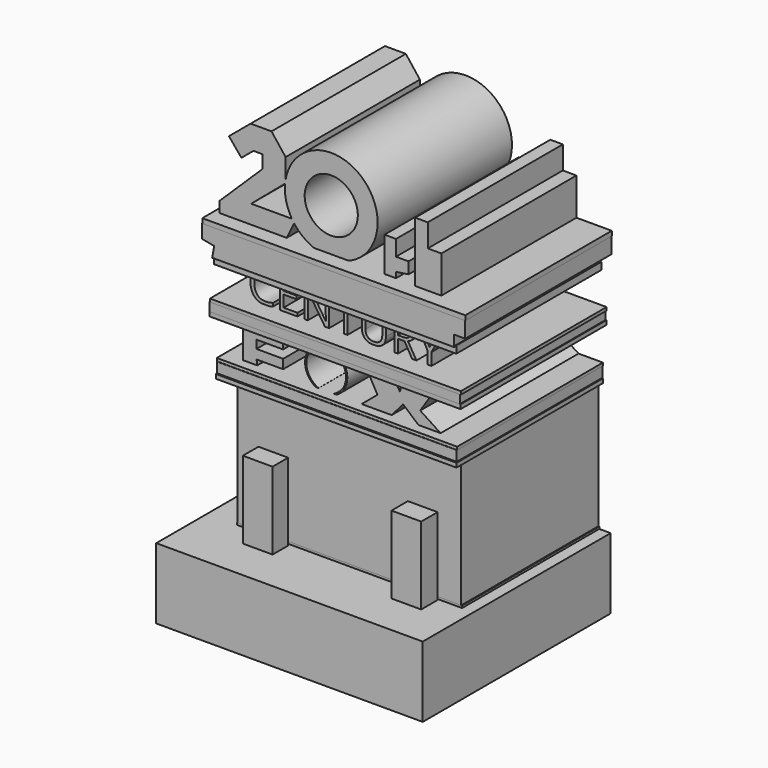
from build123d import *

# Parameters (mm, degrees)
F0_W          = 75.7836066186
F0_H          = 20.1118011028
F1_DEPTH      = 66.802
F2_W          = 63.5416395962
F2_H          = 36.7259038612
F3_DEPTH      = 48.768
F4_W          = 8.4527868312
F4_H          = 5.5380314589
F4_W_2        = 8.452789858
F4_H_2        = 5.8295056224
F5_DEPTH      = 33.528
F6_W          = 68.2052448392
F6_H          = 2.9147565365
F7_DEPTH      = 51.816
F9_DEPTH      = 49.022
F8_R          = 6.0089186636
F8_R_2        = 5.6455801804
F10_W         = 71.119999513
F10_H         = 2.623276785
F11_DEPTH     = 51.816
F12_TEXT_SIZE = 12.5496389551
F13_DEPTH     = 46.482
F15_DEPTH     = 52.07
F16_R         = 7.5582272707
F17_DEPTH     = 47.752
F19_DEPTH     = 48.006
F20_W         = 68.9278710634
F20_H         = 2.0392872393
F21_DEPTH     = 51.562
F22_W         = 71.3335052133
F22_H         = 0.8996985853
F23_DEPTH     = 51.816
F24_W         = 68.4556458145
F24_H         = 1.1931257322
F25_DEPTH     = 52.07
F26_W         = 71.3533759117
F26_H         = 1.1992175132
F27_DEPTH     = 51.816
F28_W         = 68.3553349227
F28_H         = 0.8394513279
F29_DEPTH     = 51.816
F30_W         = 64.0253070742
F30_H         = 0.6090383977
F31_DEPTH     = 48.768
F32_W         = 74.7887864709
F32_H         = 1.3311840594
F33_DEPTH     = 52.07


# Not quite as in the source:
# - Text() gives the source's letters only with a copy of the font that has no kerning and outlines rounded to 1/6400 em; it was checked with that copy


with BuildPart() as f1:
    # F0 (on Front) → F1 (new body)
    with BuildSketch(Plane.XZ):
        with Locations((10.7845906168, -32.062294893)):
            Rectangle(F0_W, F0_H)
    extrude(amount=F1_DEPTH)

    # F4 (on Top) → F5 (join)
    with BuildSketch(Plane.XY):
        with Locations((-7.724098512, -52.1930269897)):
            Rectangle(F4_W, F4_H)
        with Locations((34.5398364589, -52.0472899079)):
            Rectangle(F4_W_2, F4_H_2)
    extrude(amount=-F5_DEPTH)


with BuildPart() as f3:
    # F2 (on Front) → F3 (new body)
    with BuildSketch(Plane.XZ):
        with Locations((13.4078692645, -3.0794204213)):
            Rectangle(F2_W, F2_H)
    extrude(amount=F3_DEPTH)

    # F24 (on Front) → F25 (join)
    with BuildSketch(Plane.XZ):
        with Locations((12.2706918046, 15.4316662811)):
            Rectangle(F24_W, F24_H)
    extrude(amount=F25_DEPTH)


with BuildPart() as f7:
    # F6 (on Front) → F7 (new body)
    with BuildSketch(Plane.XZ):
        with Locations((12.2419670224, 17.6153350621)):
            Rectangle(F6_W, F6_H)
    extrude(amount=F7_DEPTH)

    # F8 (on Front) → F9 (join)
    with BuildSketch(Plane.XZ):
        with BuildLine():
            Line((-16.6140981019, 29.8573020846), (-16.6140981019, 19.3641874939))
            add(Edge.make_bspline(
                [(-12.8249172121, 21.4045159519), (-12.6287845248, 20.5804844103), (-12.1653680573, 18.6334872465), (-14.986791437, 19.0969037139), (-16.6140981019, 19.3641874939)],
                knots=[0, 0, 0, 0, 0.4232320195, 1, 1, 1, 1], degree=3))
            Line((-12.8249172121, 21.4045159519), (-5.2465572953, 21.4045159519))
            Line((-5.2465572953, 21.4045159519), (-5.2465572953, 24.0277945995))
            Line((-5.2465572953, 24.0277945995), (-12.8249172121, 24.0277945995))
            Line((-12.8249172121, 24.0277945995), (-12.8249172121, 26.359597221))
            Line((-12.8249172121, 26.359597221), (-5.2465572953, 26.359597221))
            Line((-5.2465572953, 26.359597221), (-5.2465572953, 29.8573020846))
            Line((-5.2465572953, 29.8573020846), (-16.6140981019, 29.8573020846))
        make_face()
    extrude(amount=F9_DEPTH)


with BuildPart() as f9:
    # F8 (on Front) → F9, piece 2 (new body)
    with BuildSketch(Plane.XZ):
        with Locations((6.9954101928, 25.193694979)):
            Circle(F8_R)
        with Locations((6.9954101928, 25.193694979)):
            Circle(F8_R_2, mode=Mode.SUBTRACT)
    extrude(amount=F9_DEPTH)


with BuildPart() as f9b:
    # F8 (on Front) → F9, piece 3 (new body)
    with BuildSketch(Plane.XZ):
        Polygon((25.0722425043, 31.36813441), (17.2956253181, 31.36813441), (21.5691812336, 23.7363167107), (16.6003299518, 19.5481147986), (25.2566173098, 19.5481147986), (28.8560632616, 23.7363167107), (33.729323061, 19.5481147986), (40.187170836, 19.5481147986), (33.729323061, 23.7363167107), (38.6788967572, 31.36813441), (28.8614215314, 31.36813441), (27.9869953155, 26.552970447), align=None)
    extrude(amount=F9_DEPTH)


with BuildPart() as f11:
    # F10 (on Front) → F11 (new body)
    with BuildSketch(Plane.XZ):
        with Locations((11.6590159014, 32.062294893)):
            Rectangle(F10_W, F10_H)
    extrude(amount=F11_DEPTH)


with BuildPart() as f13:
    # F12 (on Front) → F13 (new body)
    with BuildSketch(Plane.XZ):
        with Locations((-17.343884334, 34.2410169542)):
            Text('CENTURY', F12_TEXT_SIZE, font='Open Sans', text_align=(TextAlign.LEFT, TextAlign.BOTTOM))
    extrude(amount=F13_DEPTH)


with BuildPart() as f15:
    # F14 (on Front) → F15 (new body)
    with BuildSketch(Plane.XZ):
        Polygon((-22.4127210677, 47.928892076), (-22.983731702, 44.7883419693), (45.8228327334, 44.7883419693), (45.8228327334, 47.928892076), align=None)
        Polygon((-25.8798882701, 48.5592877953), (-22.4127210677, 47.928892076), (45.8228327334, 47.928892076), (48.9633828402, 47.928892076), (48.9633828402, 52.4969622493), (24.1244975477, 52.4969622493), (5.852214992, 52.4969622493), (-25.8798882701, 52.4969622493), align=None)
    extrude(amount=F15_DEPTH)

    # F16 (on Front) → F17 (join)
    with BuildSketch(Plane.XZ):
        with BuildLine():
            Line((-24.4112536311, 56.7795298994), (-24.4112536311, 52.4969622493))
            Line((-24.4112536311, 52.4969622493), (-5.6413845159, 52.9368668795))
            Line((-5.6413845159, 52.9368668795), (-3.1604204821, 58.1315330762))
            ThreePointArc((-3.1604204821, 58.1315330762), (-3.4811464405, 58.5823010843), (-3.7826858311, 59.0461231768))
            Line((-3.7826858311, 59.0461231768), (-15.3555403212, 59.0461231768))
            Line((-15.3555403212, 59.0461231768), (-5.7099537166, 67.2117787031))
            ThreePointArc((-5.7099537166, 67.2117787031), (-5.649791825, 67.7453355457), (-5.5679618381, 68.276001364))
            Line((-5.5679618381, 68.276001364), (-5.5679618381, 73.895748118))
            Line((-5.5679618381, 73.895748118), (-9.5650237054, 79.0441953886))
            Line((-9.5650237054, 79.0441953886), (-15.5091300938, 79.0441953886))
            Line((-15.5091300938, 79.0441953886), (-21.6872621161, 73.895748118))
            Line((-21.6872621161, 73.895748118), (-18.1301571429, 69.627225399))
            Line((-18.1301571429, 69.627225399), (-14.7041026503, 72.4822729826))
            Line((-14.7041026503, 72.4822729826), (-12.1345631778, 72.4822729826))
            Line((-12.1345631778, 72.4822729826), (-12.1345631778, 68.7707141042))
            Line((-12.1345631778, 68.7707141042), (-24.4112536311, 56.7795298994))
        make_face()
        with BuildLine():
            ThreePointArc((-3.7826858311, 59.0461231768), (-3.4811464405, 58.5823010843), (-3.1604204821, 58.1315330762))
            Line((-3.1604204821, 58.1315330762), (-2.7236137539, 59.0461231768))
            Line((-2.7236137539, 59.0461231768), (-3.7826858311, 59.0461231768))
        make_face()
        with BuildLine():
            Line((-2.7236137539, 59.0461231768), (-3.1604204821, 58.1315330762))
            ThreePointArc((-3.1604204821, 58.1315330762), (11.5676892115, 53.4808585189), (20.6113915013, 66.0011395812))
            ThreePointArc((20.6113915013, 66.0011395812), (8.5645945402, 79.140141992), (-5.5679618381, 68.276001364))
            Line((-5.5679618381, 68.276001364), (-5.5679618381, 67.3319846392))
            Line((-5.5679618381, 67.3319846392), (-5.7099537166, 67.2117787031))
            ThreePointArc((-5.7099537166, 67.2117787031), (-5.4129646954, 62.9716085999), (-3.7826858311, 59.0461231768))
            Line((-3.7826858311, 59.0461231768), (-2.7236137539, 59.0461231768))
        make_face()
        with Locations((7.4228774756, 66.0011395812)):
            Circle(F16_R, mode=Mode.SUBTRACT)
        with BuildLine():
            ThreePointArc((-5.5679618381, 68.276001364), (-5.649791825, 67.7453355457), (-5.7099537166, 67.2117787031))
            Line((-5.7099537166, 67.2117787031), (-5.5679618381, 67.3319846392))
            Line((-5.5679618381, 67.3319846392), (-5.5679618381, 68.276001364))
        make_face()
        Polygon((22.5655511022, 63.6258125305), (22.5655511022, 51.7492108047), (25.831617415, 51.7492108047), (25.831617415, 55.3813229625), (29.3945968151, 55.9060201049), (29.3945968151, 59.1720864177), (25.831617415, 59.1720864177), (25.831617415, 63.6258125305), align=None)
    extrude(amount=F17_DEPTH)

    # F18 (on Front) → F19 (join)
    with BuildSketch(Plane.XZ):
        Polygon((31.5024033189, 70.8890557289), (31.5024033189, 52.1659292281), (38.9322191477, 53.6518916488), (38.9322191477, 64.3508210778), (35.0687168539, 64.3508210778), (35.0687168539, 70.8890557289), align=None)
    extrude(amount=F19_DEPTH)


with BuildPart() as f21:
    # F20 (on Front) → F21 (new body)
    with BuildSketch(Plane.XZ):
        with Locations((11.5587627515, 44.0197046846)):
            Rectangle(F20_W, F20_H)
    extrude(amount=F21_DEPTH)


with BuildPart() as f23:
    # F22 (on Front) → F23 (new body)
    with BuildSketch(Plane.XZ):
        with Locations((11.8438713253, 33.7613355368)):
            Rectangle(F22_W, F22_H)
    extrude(amount=F23_DEPTH)


with BuildPart() as f27:
    # F26 (on Front) → F27 (new body)
    with BuildSketch(Plane.XZ):
        with Locations((11.761020869, 30.2809542045)):
            Rectangle(F26_W, F26_H)
    extrude(amount=F27_DEPTH)


with BuildPart() as f29:
    # F28 (on Front) → F29 (new body)
    with BuildSketch(Plane.XZ):
        with Locations((12.300667353, 19.5479663089)):
            Rectangle(F28_W, F28_H)
    extrude(amount=F29_DEPTH)


with BuildPart() as f31:
    # F30 (on Front) → F31 (new body)
    with BuildSketch(Plane.XZ):
        with Locations((13.4259639308, -21.7090854421)):
            Rectangle(F30_W, F30_H)
    extrude(amount=F31_DEPTH)


with BuildPart() as f33:
    # F32 (on Front) → F33 (new body)
    with BuildSketch(Plane.XZ):
        with Locations((11.5902535617, 53.1192477793)):
            Rectangle(F32_W, F32_H)
    extrude(amount=F33_DEPTH)


solid = Compound([f1.part, f3.part, f7.part, f9.part, f9b.part, f11.part, f13.part, f15.part, f21.part, f23.part, f27.part, f29.part, f31.part, f33.part])
